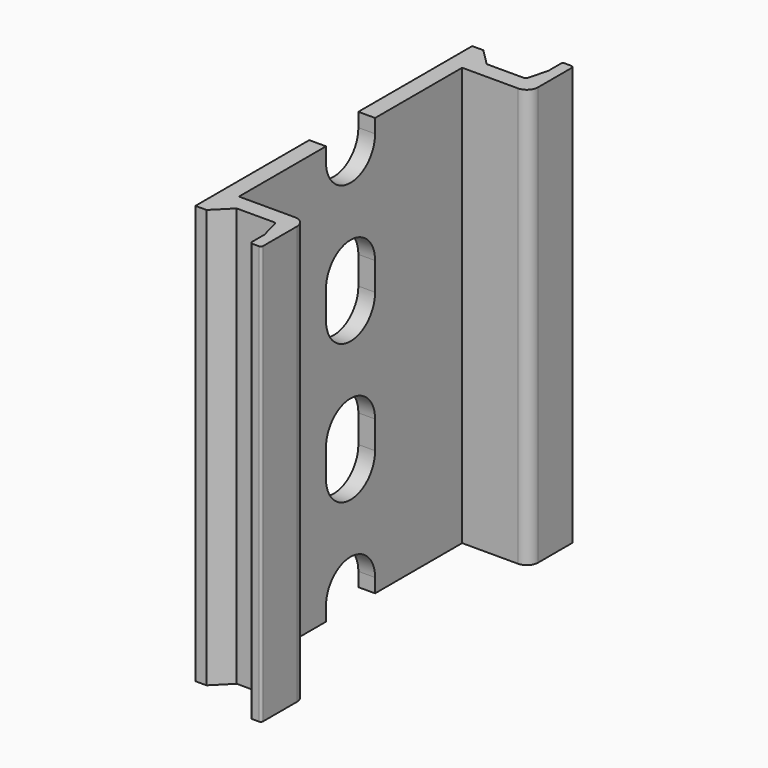
from build123d import *

# Parameters (mm, degrees)
F1_DEPTH = 37.5
F3_DEPTH = 25


# Not quite as in the source:
# - ends of sketch curves that miss each other by under 0.0002 mm in the source are joined


with BuildPart() as f1:
    # F0 (on Top) → F1 (new body)
    with BuildSketch(Plane.XY):
        with BuildLine():
            Line((-87.240451, 4.779809), (-87.240451, -5.411983))
            Line((-87.240451, -5.411983), (-87.240451, -7.720191))
            Line((-87.240451, -7.720191), (-87.240451, -17.023544))
            Line((-87.240451, -17.023544), (-87.240451, -20.220191))
            Line((-87.240451, -20.220191), (-87.240451, -23.220191))
            Line((-87.240451, -23.220191), (-86.240451, -23.220191))
            Line((-86.240451, -23.220191), (-84.740451, -21.720191))
            Line((-84.740451, -21.720191), (-81.394629, -21.720191))
            ThreePointArc((-81.394629, -21.720191), (-81.2725220613, -21.7617930975), (-81.2012141703, -21.8692920448))
            Line((-81.2012141703, -21.8692920448), (-80.747036, -23.595168))
            ThreePointArc((-80.747036, -23.595168), (-80.7421040626, -23.6204048929), (-80.740451, -23.646066))
            Line((-80.740451, -23.646066), (-80.740451, -25.020191))
            ThreePointArc((-80.740451, -25.020191), (-80.6818723562, -25.1616123562), (-80.540451, -25.220191))
            Line((-80.540451, -25.220191), (-79.940451, -25.220191))
            ThreePointArc((-79.940451, -25.220191), (-79.7990296438, -25.1616123562), (-79.740451, -25.020191))
            Line((-79.740451, -25.020191), (-79.740451, -21.220191))
            ThreePointArc((-79.740451, -21.220191), (-80.0333442188, -20.5130842188), (-80.740451, -20.220191))
            Line((-80.740451, -20.220191), (-85.740451, -20.220191))
            Line((-85.740451, -20.220191), (-85.740451, -7.720191))
            Line((-85.740451, -7.720191), (-85.740451, 4.779809))
            Line((-85.740451, 4.779809), (-80.740451, 4.779809))
            ThreePointArc((-80.740451, 4.779809), (-80.0333442188, 5.0727022188), (-79.740451, 5.779809))
            Line((-79.740451, 5.779809), (-79.740451, 9.579809))
            ThreePointArc((-79.740451, 9.579809), (-79.7990296438, 9.7212303562), (-79.940451, 9.779809))
            Line((-79.940451, 9.779809), (-80.540451, 9.779809))
            ThreePointArc((-80.540451, 9.779809), (-80.6818723562, 9.7212303562), (-80.740451, 9.579809))
            Line((-80.740451, 9.579809), (-80.740451, 8.205684))
            ThreePointArc((-80.740451, 8.205684), (-80.7421040626, 8.1800228929), (-80.7470359242, 8.15478598))
            Line((-80.7470359242, 8.15478598), (-81.201214, 6.42891))
            ThreePointArc((-81.201214, 6.42891), (-81.2725220613, 6.3214110975), (-81.394629, 6.279809))
            Line((-81.394629, 6.279809), (-84.740451, 6.279809))
            Line((-84.740451, 6.279809), (-86.240451, 7.779809))
            Line((-86.240451, 7.779809), (-87.240451, 7.779809))
            Line((-87.240451, 7.779809), (-87.240451, 4.779809))
        make_face()
    extrude(amount=F1_DEPTH)

    # F2 (on face) → F3 (cut)
    with BuildSketch(Plane.YZ.offset(-85.740451)):
        with BuildLine():
            ThreePointArc((-10.470191, 23.75), (-7.720191, 21), (-4.970191, 23.75))
            Line((-4.970191, 23.75), (-4.970191, 26.25))
            ThreePointArc((-4.970191, 26.25), (-7.720191, 29), (-10.470191, 26.25))
            Line((-10.470191, 26.25), (-10.470191, 23.75))
        make_face()
        with BuildLine():
            Line((-4.970191, 11.25), (-4.970191, 13.75))
            ThreePointArc((-4.970191, 13.75), (-7.720191, 16.5), (-10.470191, 13.75))
            Line((-10.470191, 13.75), (-10.470191, 11.25))
            ThreePointArc((-10.470191, 11.25), (-7.720191, 8.5), (-4.970191, 11.25))
        make_face()
        with BuildLine():
            Line((-4.970191, -1.25), (-4.970191, 1.25))
            ThreePointArc((-4.970191, 1.25), (-7.720191, 4), (-10.470191, 1.25))
            Line((-10.470191, 1.25), (-10.470191, -1.25))
            ThreePointArc((-10.470191, -1.25), (-7.720191, -4), (-4.970191, -1.25))
        make_face()
        with BuildLine():
            Line((-4.970191, 36.25), (-4.970191, 38.75))
            ThreePointArc((-4.970191, 38.75), (-7.720191, 41.5), (-10.470191, 38.75))
            Line((-10.470191, 38.75), (-10.470191, 36.25))
            ThreePointArc((-10.470191, 36.25), (-7.720191, 33.5), (-4.970191, 36.25))
        make_face()
    extrude(amount=-F3_DEPTH, mode=Mode.SUBTRACT)


solid = f1.part
